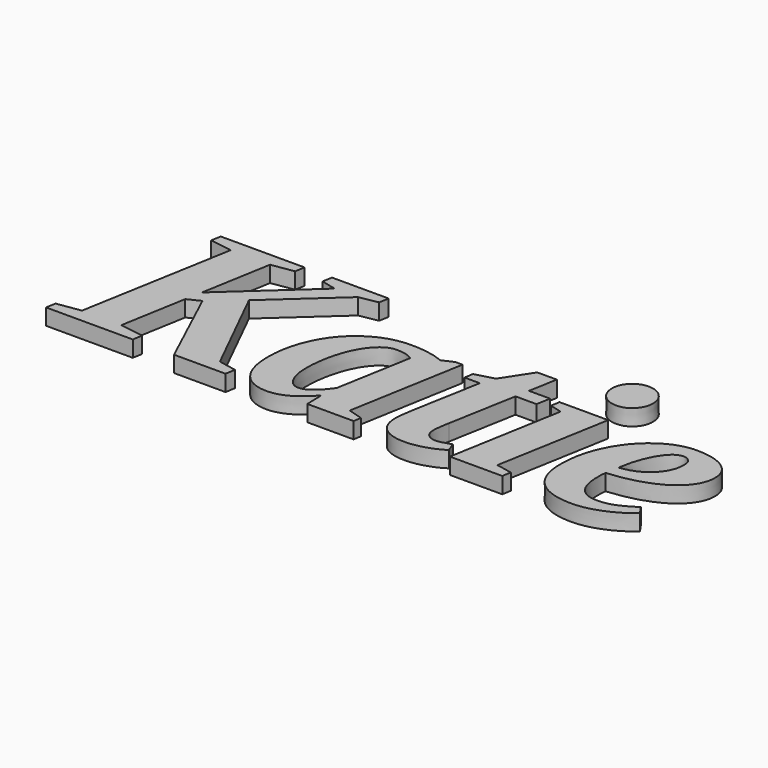
from build123d import *

# Parameters (mm, degrees)
F0_TEXT_SIZE = 50.6687838222
F1_DEPTH     = 3


# Not quite as in the source:
# - Text() gives the source's letters only with a copy of the font that has no kerning and outlines rounded to 1/6400 em; it was checked with that copy


with BuildPart() as f1:
    # F0 (on Top) → F1 (new body)
    with BuildSketch(Plane.XY):
        with Locations((-55.8113195002, 6.704044994)):
            Text('Katie', F0_TEXT_SIZE, font='Tinos', font_style=FontStyle.BOLDITALIC, text_align=(TextAlign.LEFT, TextAlign.BOTTOM))
    extrude(amount=F1_DEPTH)


solid = f1.part
